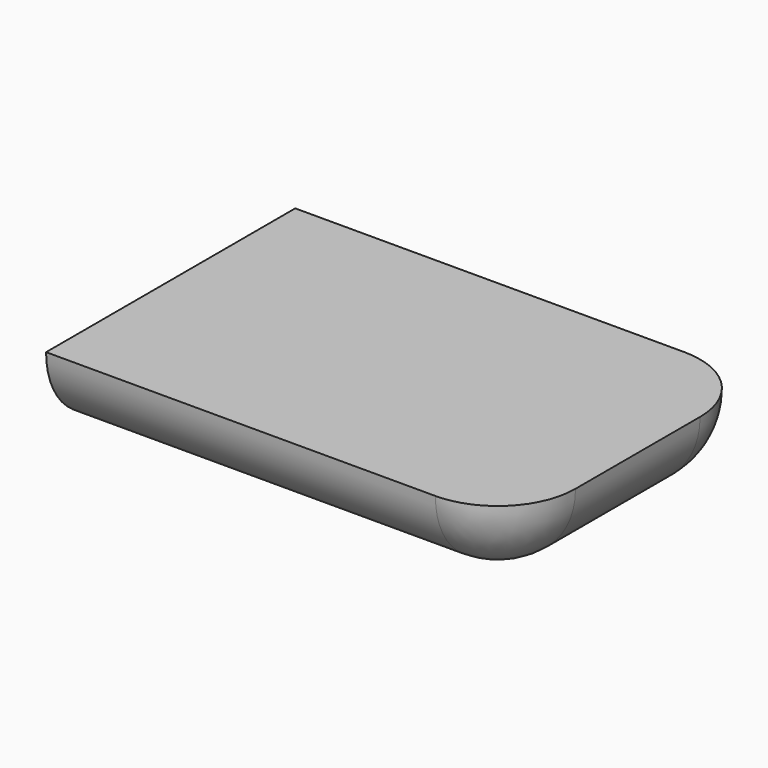
from build123d import *

# Parameters (mm, degrees)
F0_W     = 127
F0_H     = 25.4
F1_DEPTH = 25.4
F2_DEPTH = 76.2
F3_R     = 25.39999
F4_R     = 25.39999


# Not quite as in the source:
# - a fillet or chamfer is up to 0.001 mm smaller than in the source, because OpenCascade refuses the exact size


with BuildPart() as f1:
    # F0 (on Front) → F1 (new body)
    with BuildSketch(Plane.XZ):
        with Locations((-27.0015653223, 9.674326013)):
            Rectangle(F0_W, F0_H)
        with BuildLine():
            Line((61.8984346777, 22.374326013), (36.4984346777, 22.374326013))
            Line((36.4984346777, 22.374326013), (36.4984346777, -3.025673987))
            ThreePointArc((36.4984346777, -3.025673987), (54.4589469199, 4.4138137708), (61.8984346777, 22.374326013))
        make_face()
    extrude(amount=F1_DEPTH)

    # F2 (add): a face of the model
    f2_faces = [f1.faces().sort_by_distance(p)[0] for p in [
        (-16.9176526174, -25.4, 9.9349632182),
    ]]
    extrude(f2_faces, amount=F2_DEPTH)

    # F3 (radius 25.4 in the source; OpenCascade refuses exactly that, so slightly less here)
    f3_edges = [f1.edges().sort_by_distance(p)[0] for p in [
        (-27.001565, -101.6, -3.025674),
    ]]
    fillet(f3_edges, radius=F3_R)

    # F4 (radius 25.4 in the source; OpenCascade refuses exactly that, so slightly less here)
    f4_edges = [f1.edges().sort_by_distance(p)[0] for p in [
        (-27.001565, 0, -3.025674),
    ]]
    fillet(f4_edges, radius=F4_R)


solid = f1.part
